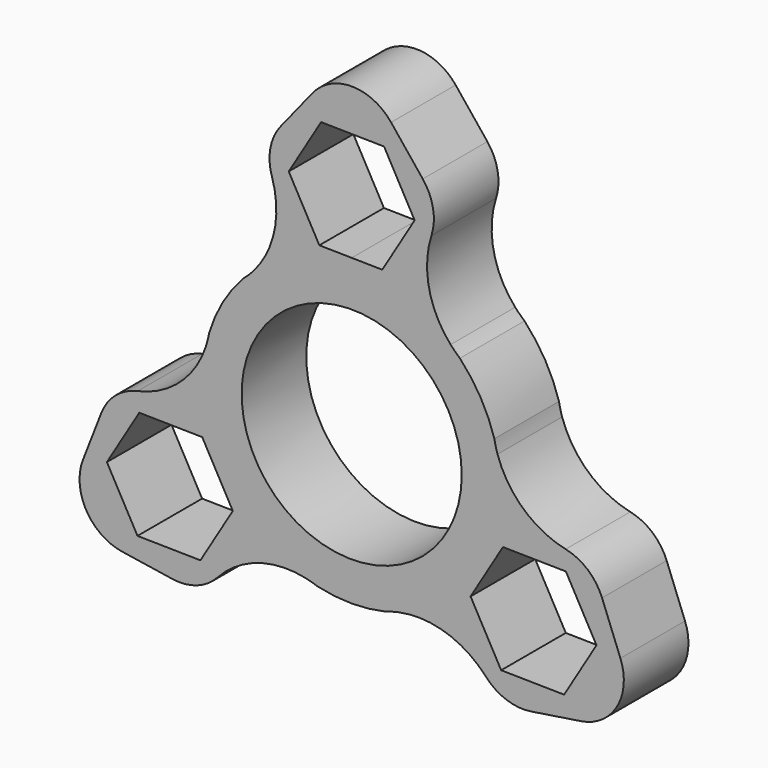
from build123d import *

# Parameters (mm, degrees)
F0_R     = 10.9
F1_DEPTH = 8
F2_R     = 5


with BuildPart() as f1:
    # F0 (on Front) → F1 (new body)
    with BuildSketch(Plane.XZ):
        with BuildLine():
            ThreePointArc((-4.6474292299, -13.9936443391), (-12.7697106566, -7.372595885), (-14.4425661041, 2.9720303942))
            ThreePointArc((-14.4425661041, 2.9720303942), (-17.9890829323, -1.7394577094), (-23.6744608764, -3.305465179))
            Line((-23.6744608764, -3.305465179), (-26.6141080798, -10.8626586404))
            ThreePointArc((-26.6141080798, -10.8626586404), (-26.2843656104, -15.1752855606), (-22.7143923751, -17.617164376))
            Line((-22.7143923751, -17.617164376), (-14.6998472546, -18.8499519504))
            ThreePointArc((-14.6998472546, -18.8499519504), (-10.5009560313, -14.7092739554), (-4.6474292299, -13.9936443391))
        make_face()
        Polygon((-21.2154018643, -15.7464514283), (-24.2445278885, -10.2962775292), (-21.039101849, -4.9478904915), (-14.8045497853, -5.0496773528), (-11.7754237611, -10.4998512519), (-14.9808498006, -15.8482382896), align=None, mode=Mode.SUBTRACT)
        with BuildLine():
            ThreePointArc((9.7951368743, 11.0216139449), (5.2395070905, 13.7828968575), (0, 14.7451917701))
            ThreePointArc((0, 14.7451917701), (-5.2395070905, 13.7828968575), (-9.7951368743, 11.0216139449))
            ThreePointArc((-9.7951368743, 11.0216139449), (-10.2405850834, 10.5580719376), (-10.7175072848, 10.1269797045))
            ThreePointArc((-10.7175072848, 10.1269797045), (-12.7697106566, 7.372595885), (-14.1289753301, 4.2181437217))
            ThreePointArc((-14.1289753301, 4.2181437217), (-14.2638510546, 3.5895708631), (-14.4425661041, 2.9720303942))
            ThreePointArc((-14.4425661041, 2.9720303942), (-12.7697106566, -7.372595885), (-4.6474292299, -13.9936443391))
            ThreePointArc((-4.6474292299, -13.9936443391), (-4.0232659712, -14.1476428006), (-3.4114680453, -14.3451234262))
            ThreePointArc((-3.4114680453, -14.3451234262), (0, -14.7451917701), (3.4114680453, -14.3451234262))
            ThreePointArc((3.4114680453, -14.3451234262), (4.0232659712, -14.1476428006), (4.6474292299, -13.9936443391))
            ThreePointArc((4.6474292299, -13.9936443391), (11.9571718138, -8.6282514191), (14.7451917701, 0))
            ThreePointArc((14.7451917701, 0), (14.6693402577, 1.4936990123), (14.4425661041, 2.9720303942))
            ThreePointArc((14.4425661041, 2.9720303942), (14.2638510546, 3.5895708631), (14.1289753301, 4.2181437217))
            ThreePointArc((14.1289753301, 4.2181437217), (12.7697106566, 7.372595885), (10.7175072848, 10.1269797045))
            ThreePointArc((10.7175072848, 10.1269797045), (10.2405850834, 10.5580719376), (9.7951368743, 11.0216139449))
        make_face()
        Circle(F0_R, mode=Mode.SUBTRACT)
        with BuildLine():
            ThreePointArc((23.6744608764, -3.305465179), (17.9890829323, -1.7394577094), (14.4425661041, 2.9720303942))
            ThreePointArc((14.4425661041, 2.9720303942), (14.6693402577, 1.4936990123), (14.7451917701, 0))
            ThreePointArc((14.7451917701, 0), (11.9571718138, -8.6282514191), (4.6474292299, -13.9936443391))
            ThreePointArc((4.6474292299, -13.9936443391), (10.5009560313, -14.7092739554), (14.6998472546, -18.8499519504))
            Line((14.6998472546, -18.8499519504), (22.7143923751, -17.617164376))
            ThreePointArc((22.7143923751, -17.617164376), (26.2843656104, -15.1752855606), (26.6141080798, -10.8626586404))
            Line((26.6141080798, -10.8626586404), (23.6744608764, -3.305465179))
        make_face()
        Polygon((24.2445278885, -10.4998512519), (21.039101849, -15.8482382896), (14.8045497853, -15.7464514283), (11.7754237611, -10.2962775292), (14.9808498006, -4.9478904915), (21.2154018643, -5.0496773528), align=None, mode=Mode.SUBTRACT)
        with BuildLine():
            ThreePointArc((-9.7951368743, 11.0216139449), (-5.2395070905, 13.7828968575), (0, 14.7451917701))
            ThreePointArc((0, 14.7451917701), (5.2395070905, 13.7828968575), (9.7951368743, 11.0216139449))
            ThreePointArc((9.7951368743, 11.0216139449), (7.488126901, 16.4487316648), (8.9746136218, 22.1554171294))
            Line((8.9746136218, 22.1554171294), (3.8997157047, 28.4798230164))
            ThreePointArc((3.8997157047, 28.4798230164), (0, 30.3505711213), (-3.8997157047, 28.4798230164))
            Line((-3.8997157047, 28.4798230164), (-8.9746136218, 22.1554171294))
            ThreePointArc((-8.9746136218, 22.1554171294), (-7.488126901, 16.4487316648), (-9.7951368743, 11.0216139449))
        make_face()
        Polygon((3.0291260242, 15.3459548821), (0, 15.3954091536), (-3.2054260395, 15.4477417434), (-6.2345520637, 20.8979156424), (-3.0291260242, 26.2463026801), (3.2054260395, 26.1445158188), (6.2345520637, 20.6943419198), align=None, mode=Mode.SUBTRACT)
    extrude(amount=F1_DEPTH)

    # F2
    f2_edges = [f1.edges().sort_by_distance(p)[0] for p in [
        (-23.674461, -4, -3.305465),
        (-14.699847, -4, -18.849952),
        (14.699847, -4, -18.849952),
        (23.674461, -4, -3.305465),
        (8.974614, -4, 22.155417),
        (-8.974614, -4, 22.155417),
    ]]
    fillet(f2_edges, radius=F2_R)


solid = f1.part
